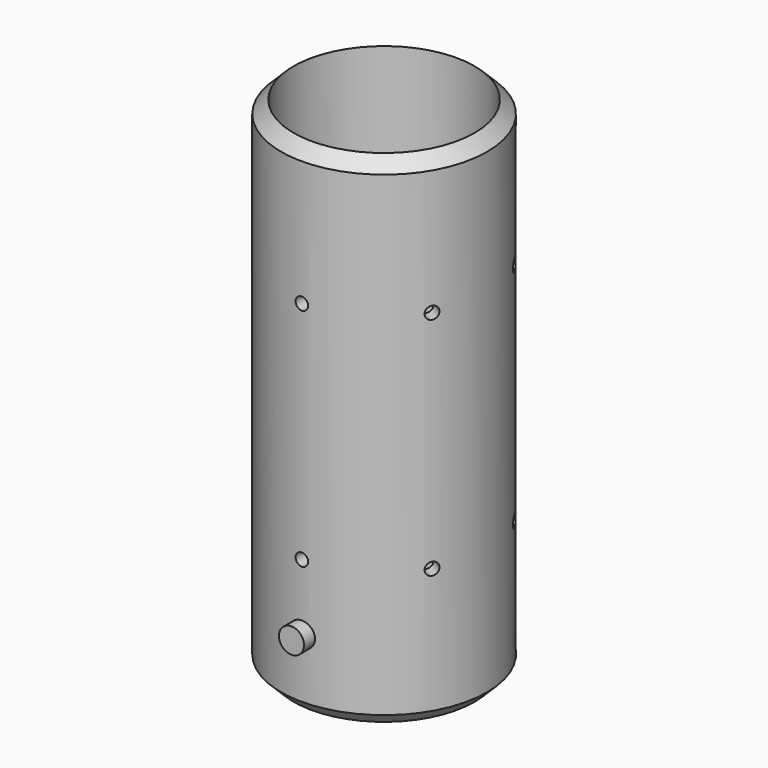
from build123d import *

# Parameters (mm, degrees)
F3_R            = 2.54
F4_DEPTH        = 23.495
F5_DEPTH        = 16.51
F6_R            = 1.27
F7_DEPTH        = 50.8
F7_COPIES_COUNT = 3
F7_COPIES_ANGLE = 120
F8_R            = 1.27
F9_DEPTH        = 63.5
F9_COPIES_COUNT = 3
F9_COPIES_ANGLE = 120


# Not quite as in the source:
# - a pattern or mirror of a feature is missing from the dataset's text; its kind, count and spacing are read off the source's solid


with BuildPart() as f2:
    # F0 (on Front) → F2 (revolve)
    with BuildSketch(Plane.XZ):
        Polygon((20.8915, 71.824210396), (18.3515, 74.364210396), (18.3515, -27.235789604), (20.8915, -24.695789604), align=None)
    revolve(axis=Axis((0, 0, 23.4525538981), (0, 0, -1)))

    # F6 (on Front) → F7 (cut, symmetric)
    with BuildSketch(Plane.XZ):
        with Locations((0, 46.424210396)):
            Circle(F6_R)
    f7 = extrude(amount=F7_DEPTH, both=True, mode=Mode.SUBTRACT)

    # F7_copies: F7 ×3 about axis
    f7_copies_axis = Axis((0, 0, 0), (0, 0, 1))
    for i in range(1, F7_COPIES_COUNT):
        add(f7.rotate(f7_copies_axis, i * F7_COPIES_ANGLE / (F7_COPIES_COUNT - 1)), mode=Mode.SUBTRACT)

    # F8 (on Front) → F9 (cut, symmetric)
    with BuildSketch(Plane.XZ):
        with Locations((0, 0.704210396)):
            Circle(F8_R)
    f9 = extrude(amount=F9_DEPTH, both=True, mode=Mode.SUBTRACT)

    # F9_copies: F9 ×3 about axis
    f9_copies_axis = Axis((0, 0, 0), (0, 0, 1))
    for i in range(1, F9_COPIES_COUNT):
        add(f9.rotate(f9_copies_axis, i * F9_COPIES_ANGLE / (F9_COPIES_COUNT - 1)), mode=Mode.SUBTRACT)


with BuildPart() as f4:
    # F3 (on Front) → F4 (new body, symmetric)
    with BuildSketch(Plane.XZ):
        with Locations((0, -12.7)):
            Circle(F3_R)
    extrude(amount=F4_DEPTH, both=True)

    # F3 (on Front) → F5 (cut, symmetric)
    with BuildSketch(Plane.XZ):
        with Locations((0, -12.7)):
            Circle(F3_R)
    extrude(amount=F5_DEPTH, both=True, mode=Mode.SUBTRACT)


solid = Compound([f2.part, f4.part])
